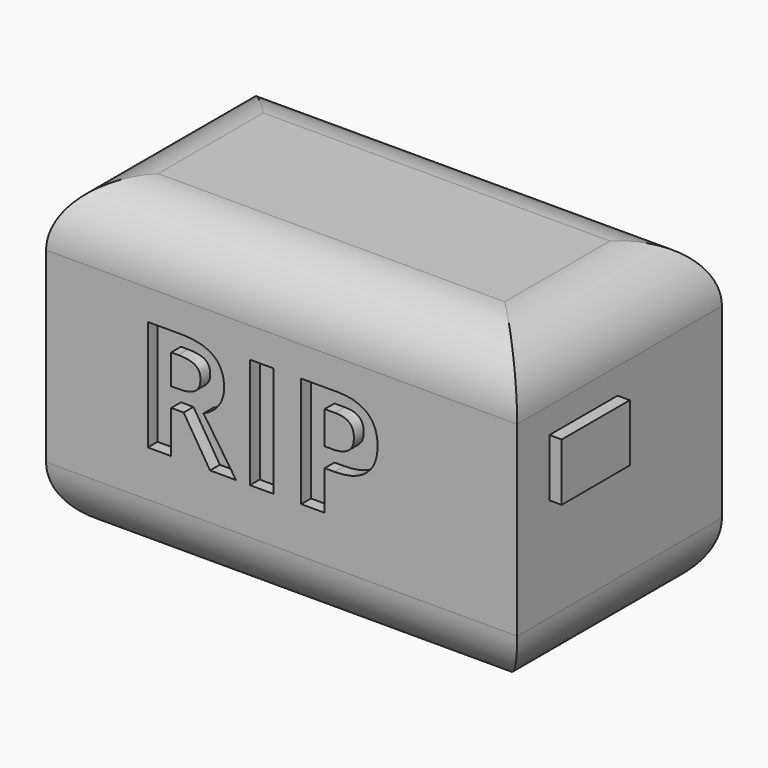
from build123d import *

# Parameters (mm, degrees)
F0_W         = 38.4787991643
F0_H         = 20.9043454379
F1_DEPTH     = 25.4
F2_R         = 5.08
F3_TEXT_SIZE = 12.6445096814
F4_DEPTH     = 1
F6_DEPTH     = 1


# Not quite as in the source:
# - Text() gives the source's letters only with a copy of the font that has no kerning and outlines rounded to 1/6400 em; it was checked with that copy


with BuildPart() as f1:
    # F0 (on Top) → F1 (new body)
    with BuildSketch(Plane.XY):
        with Locations((-42.9186597466, 29.9690635875)):
            Rectangle(F0_W, F0_H)
    extrude(amount=F1_DEPTH)

    # F2
    f2_edges = [f1.edges().sort_by_distance(p)[0] for p in [
        (-42.91866, 19.516891, 25.4),
        (-42.91866, 40.421236, 25.4),
        (-62.158059, 29.969064, 0),
        (-23.67926, 29.969064, 0),
        (-42.91866, 19.516891, 0),
        (-42.91866, 40.421236, 0),
        (-62.158059, 29.969064, 25.4),
        (-23.67926, 29.969064, 25.4),
    ]]
    fillet(f2_edges, radius=F2_R)

    # F3 (on face) → F4 (cut)
    with BuildSketch(Plane.XZ.offset(-19.5168908685)):
        with Locations((-54.9884401262, 8.8309254497)):
            Text('RIP', F3_TEXT_SIZE, font='Open Sans', font_style=FontStyle.BOLD, text_align=(TextAlign.LEFT, TextAlign.BOTTOM))
    extrude(amount=-F4_DEPTH, mode=Mode.SUBTRACT)

    # F5 (on face) → F6 (join)
    with BuildSketch(Plane.YZ.offset(-23.6792601645)):
        Polygon((22.8123832494, 13.5003123432), (29.7649204731, 13.5164055973), (29.7649204731, 18.199712038), (22.8123832494, 18.199712038), align=None)
    extrude(amount=F6_DEPTH)


solid = f1.part
